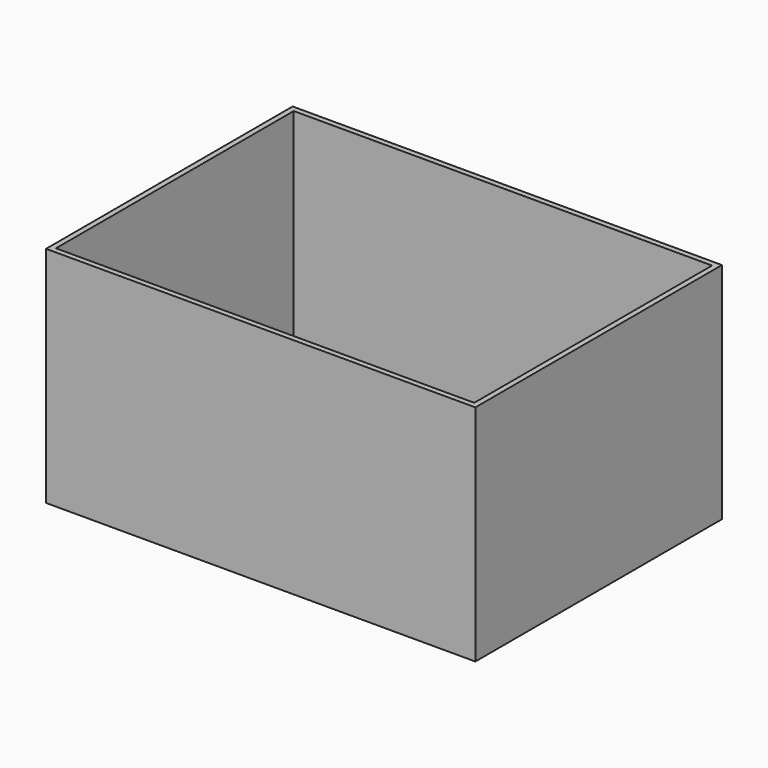
from build123d import *

# Parameters (mm, degrees)
F1_DEPTH = 311.15
F2_T     = -7.62


# Not quite as in the source:
# - a feature names something its author has since deleted; it is built from what else it names


with BuildPart() as f1:
    # F0 (on Top) → F1 (new body)
    with BuildSketch(Plane.XY):
        Polygon((342.2408003828, -255.094484383), (342.2408003828, 173.456788063), (-254.6591996172, 173.456788063), (-254.6591996172, -197.8495568037), (-254.6591996172, -255.094484383), (334.2911142349, -255.094484383), align=None)
    extrude(amount=F1_DEPTH)

    # F2
    f2_openings = [f1.faces().sort_by_distance(p)[0] for p in [
        (43.7908, -40.818848, 311.15),
    ]]
    offset(amount=F2_T, openings=f2_openings)


solid = f1.part
